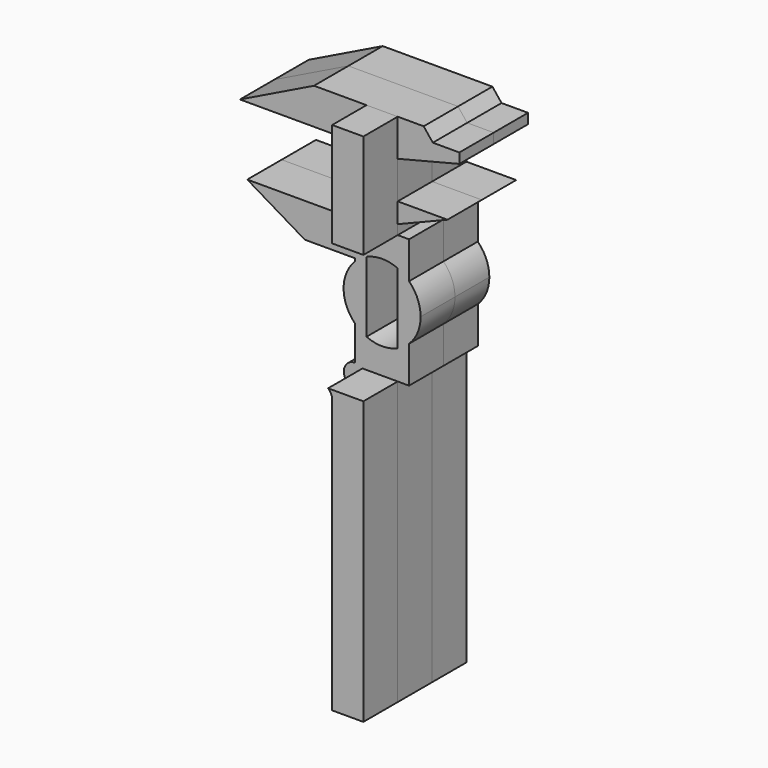
from build123d import *

# Parameters (mm, degrees)
F1_DEPTH  = 25.4
F1_FACE_W = 9.2242108179
F1_FACE_H = 30.834726283
F2_DEPTH  = 12.7
F3_DEPTH  = 12.7


with BuildPart() as f1:
    # F0 (on Front) → F1 (new body)
    with BuildSketch(Plane.XZ):
        with BuildLine():
            Line((-7.9663358629, 7.265273717), (-5.8154628601, 7.265273717))
            ThreePointArc((-5.8154628601, 7.265273717), (-6.822299412, 7.8445429389), (-7.9663358629, 8.0456729287))
            Line((-7.9663358629, 8.0456729287), (-7.9663358629, 7.265273717))
        make_face()
    extrude(amount=F1_DEPTH)


with BuildPart() as f1b:
    # F0 (on Front) → F1, piece 2 (new body)
    with BuildSketch(Plane.XZ):
        with BuildLine():
            Line((-4.6121054089, 4.6914424747), (-4.6121054089, 7.265273717))
            Line((-4.6121054089, 7.265273717), (-5.8154628601, 7.265273717))
            ThreePointArc((-5.8154628601, 7.265273717), (-4.9278012106, 6.1120652624), (-4.6121054089, 4.6914424747))
        make_face()
        Polygon((4.6121054089, 7.265273717), (-4.6121054089, 7.265273717), (-4.6121054089, 4.6914424747), (-4.6121054089, -76.2), (4.6121054089, -76.2), align=None)
    extrude(amount=F1_DEPTH)


with BuildPart() as f1c:
    # F0 (on Front) → F1, piece 3 (new body)
    with BuildSketch(Plane.XZ):
        Polygon((4.6121054089, 65.2381628752), (4.6121054089, 76.2), (-4.6121054089, 76.2), (-4.6121054089, 65.5084699392), (-4.6121054089, 45.365273717), (4.6121054089, 45.365273717), (4.6121054089, 48.2094027102), (4.6121054089, 54.1559569538), align=None)
    extrude(amount=F1_DEPTH)


with BuildPart() as f2:
    # F0 (on Front) + F1_face (on face) → F2 (new body)
    with BuildSketch(Plane.XZ):
        Polygon((4.6121054089, 65.2381628752), (4.6121054089, 76.2), (-4.6121054089, 76.2), (-4.6121054089, 65.5084699392), (-4.6121054089, 45.365273717), (4.6121054089, 45.365273717), (4.6121054089, 48.2094027102), (4.6121054089, 54.1559569538), align=None)
        Polygon((12.2911036015, 76.2), (4.6121054089, 76.2), (4.6121054089, 65.2381628752), (22.8327196091, 69.8332339525), (22.8327196091, 72.8065147996), (17.9673600942, 72.8065147996), (14.9940820411, 72.8065147996), align=None)
        Polygon((-4.6121054089, 65.5084699392), (-4.6121054089, 76.2), (-20.144643262, 76.2), (-42.0387722552, 65.5084699392), align=None)
        Polygon((19.3188488483, 54.1559569538), (4.6121054089, 54.1559569538), (4.6121054089, 48.2094027102), align=None)
        with BuildLine():
            Line((4.6121054089, 45.365273717), (-4.6121054089, 45.365273717))
            Line((-4.6121054089, 45.365273717), (-4.6121054089, 36.7256611241))
            ThreePointArc((-4.6121054089, 36.7256611241), (0, 37.7015673313), (4.6121054089, 36.7256611241))
            Line((4.6121054089, 36.7256611241), (4.6121054089, 45.365273717))
        make_face()
        with BuildLine():
            Line((-4.6121054089, 36.7256611241), (-4.6121054089, 45.365273717))
            Line((-4.6121054089, 45.365273717), (-7.9663358629, 45.365273717))
            Line((-7.9663358629, 45.365273717), (-7.9663358629, 35.2351032197))
            Line((-7.9663358629, 35.2351032197), (-7.9663358629, 34.450700884))
            ThreePointArc((-7.9663358629, 34.450700884), (-6.3912563108, 35.7386237073), (-4.6121054089, 36.7256611241))
        make_face()
        with BuildLine():
            Line((-4.6121054089, 15.90488631), (-4.6121054089, 36.7256611241))
            ThreePointArc((-4.6121054089, 36.7256611241), (-6.3912563108, 35.7386237073), (-7.9663358629, 34.450700884))
            Line((-7.9663358629, 34.450700884), (-7.9663358629, 18.1798465501))
            ThreePointArc((-7.9663358629, 18.1798465501), (-6.3912563108, 16.8919237268), (-4.6121054089, 15.90488631))
        make_face()
        with BuildLine():
            Line((7.9663358629, 45.365273717), (4.6121054089, 45.365273717))
            Line((4.6121054089, 45.365273717), (4.6121054089, 36.7256611241))
            ThreePointArc((4.6121054089, 36.7256611241), (6.3912563108, 35.7386237073), (7.9663358629, 34.450700884))
            Line((7.9663358629, 34.450700884), (7.9663358629, 45.365273717))
        make_face()
        Polygon((-7.9663358629, 35.2351032197), (-7.9663358629, 45.365273717), (-39.8763902485, 45.365273717), (-22.847622633, 35.2351032197), align=None)
        with BuildLine():
            ThreePointArc((4.6121054089, 15.90488631), (0, 14.9289801028), (-4.6121054089, 15.90488631))
            Line((-4.6121054089, 15.90488631), (-4.6121054089, 7.265273717))
            Line((-4.6121054089, 7.265273717), (4.6121054089, 7.265273717))
            Line((4.6121054089, 7.265273717), (4.6121054089, 15.90488631))
        make_face()
        with BuildLine():
            Line((-4.6121054089, 7.265273717), (-4.6121054089, 15.90488631))
            ThreePointArc((-4.6121054089, 15.90488631), (-6.3912563108, 16.8919237268), (-7.9663358629, 18.1798465501))
            Line((-7.9663358629, 18.1798465501), (-7.9663358629, 8.0456729287))
            ThreePointArc((-7.9663358629, 8.0456729287), (-6.822299412, 7.8445429389), (-5.8154628601, 7.265273717))
            Line((-5.8154628601, 7.265273717), (-4.6121054089, 7.265273717))
        make_face()
        with BuildLine():
            ThreePointArc((7.9663358629, 34.450700884), (6.3912563108, 35.7386237073), (4.6121054089, 36.7256611241))
            Line((4.6121054089, 36.7256611241), (4.6121054089, 15.90488631))
            ThreePointArc((4.6121054089, 15.90488631), (6.3912563108, 16.8919237268), (7.9663358629, 18.1798465501))
            Line((7.9663358629, 18.1798465501), (7.9663358629, 34.450700884))
        make_face()
        with BuildLine():
            Line((-7.9663358629, 18.1798465501), (-7.9663358629, 34.450700884))
            ThreePointArc((-7.9663358629, 34.450700884), (-11.3862936142, 26.315273717), (-7.9663358629, 18.1798465501))
        make_face()
        Polygon((4.6121054089, 7.265273717), (-4.6121054089, 7.265273717), (-4.6121054089, 4.6914424747), (-4.6121054089, -76.2), (4.6121054089, -76.2), align=None)
        with BuildLine():
            Line((-4.6121054089, 4.6914424747), (-4.6121054089, 7.265273717))
            Line((-4.6121054089, 7.265273717), (-5.8154628601, 7.265273717))
            ThreePointArc((-5.8154628601, 7.265273717), (-4.9278012106, 6.1120652624), (-4.6121054089, 4.6914424747))
        make_face()
        with BuildLine():
            ThreePointArc((7.9663358629, 18.1798465501), (6.3912563108, 16.8919237268), (4.6121054089, 15.90488631))
            Line((4.6121054089, 15.90488631), (4.6121054089, 7.265273717))
            Line((4.6121054089, 7.265273717), (7.9663358629, 7.265273717))
            Line((7.9663358629, 7.265273717), (7.9663358629, 18.1798465501))
        make_face()
        with BuildLine():
            ThreePointArc((11.3862936142, 26.315273717), (10.4965404166, 30.7277924482), (7.9663358629, 34.450700884))
            Line((7.9663358629, 34.450700884), (7.9663358629, 18.1798465501))
            ThreePointArc((7.9663358629, 18.1798465501), (10.4965404166, 21.9027549859), (11.3862936142, 26.315273717))
        make_face()
        with BuildLine():
            ThreePointArc((-7.9663358629, 8.0456729287), (-10.3381349625, 2.3196433751), (-4.6121054089, 4.6914424747))
            ThreePointArc((-4.6121054089, 4.6914424747), (-4.9278012106, 6.1120652624), (-5.8154628601, 7.265273717))
            Line((-5.8154628601, 7.265273717), (-7.9663358629, 7.265273717))
            Line((-7.9663358629, 7.265273717), (-7.9663358629, 8.0456729287))
        make_face()
        with BuildLine():
            Line((-7.9663358629, 7.265273717), (-5.8154628601, 7.265273717))
            ThreePointArc((-5.8154628601, 7.265273717), (-6.822299412, 7.8445429389), (-7.9663358629, 8.0456729287))
            Line((-7.9663358629, 8.0456729287), (-7.9663358629, 7.265273717))
        make_face()
    with BuildSketch(Plane(origin=(-0.00607725, -25.4, -34.4169717723), x_dir=(1, 0, 0), z_dir=(0, -1, 0))):
        with BuildLine():
            ThreePointArc((-5.8093856101, 41.6822454894), (-4.9217239606, 40.5290370347), (-4.606028159, 39.1084142471))
            Line((-4.606028159, 39.1084142471), (-4.606028159, -41.7830282277))
            Line((-4.606028159, -41.7830282277), (4.6181826589, -41.7830282277))
            Line((4.6181826589, -41.7830282277), (4.6181826589, 41.6822454894))
            Line((4.6181826589, 41.6822454894), (-5.8093856101, 41.6822454894))
        make_face()
        with Locations((0.00607725, 95.1996086309)):
            Rectangle(F1_FACE_W, F1_FACE_H)
    extrude(amount=F2_DEPTH)


with BuildPart() as f3:
    # F3 (new): a face of the model
    f3_faces = [f2.part.faces().sort_by_distance(p)[0] for p in [
        (-6.3100125111, -12.7, 13.1127597394),
    ]]
    extrude(f3_faces, amount=F3_DEPTH)


solid = Compound([f1.part, f1b.part, f1c.part, f2.part, f3.part])
